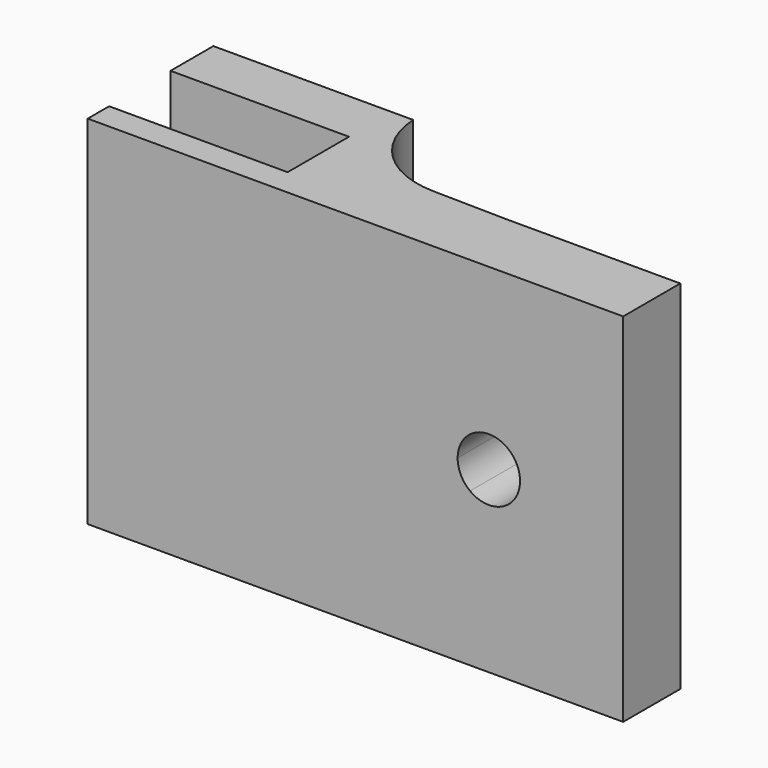
from build123d import *

# Parameters (mm, degrees)
F1_DEPTH    = 20
F2_T1_DEPTH = 20
F4_DEPTH    = 25


# Not quite as in the source:
# - a fillet or chamfer that OpenCascade refuses, or shapes differently, is made with other operations: its cross-section is extruded or revolved along the edge and cut away or added


with BuildPart() as f1:
    # F0 (on Top) → F1 (new body)
    with BuildSketch(Plane.XY):
        Polygon((-30, 0), (0, 0), (0, 1.4936865721), (0, 2.9873731442), (0, 4), (-9.7294932483, 4), (-18.8047308475, 4.1669379548), (-18.8047308475, 8.8), (-30, 8.8), (-30, 5.8), (-20, 5.8), (-20, 1.5), (-30, 1.5), align=None)
    extrude(amount=F1_DEPTH)

    # F2: fillet of radius 5 on 2 edges, made by hand

    # F2_s2 → F2_t1 (join)
    with BuildSketch(Plane.XY):
        with BuildLine():
            ThreePointArc((-9.7754687943, 4.0008457149), (-9.7294913038, 4.0002114332), (-9.6835099246, 4))
            Line((-9.6835099246, 4), (-9.7294932483, 4))
            Line((-9.7294932483, 4), (-9.7754687943, 4.0008457149))
        make_face()
        with BuildLine():
            ThreePointArc((-18.8047308475, 8.8), (-17.2821914607, 5.4759203381), (-13.904310341, 4.0767952816))
            Line((-13.904310341, 4.0767952816), (-18.8047308475, 4.1669379548))
            Line((-18.8047308475, 4.1669379548), (-18.8047308475, 8.8))
        make_face()
    extrude(amount=F2_T1_DEPTH)

    # F3 (on face) → F4 (cut)
    with BuildSketch(Plane(origin=(0, 4, 0), x_dir=(-1, 0, 0), z_dir=(0, 1, 0))):
        with BuildLine():
            Line((6.4737138013, 11.3982501667), (7.5260428712, 10))
            Line((7.5260428712, 10), (8.5783719411, 11.3982501667))
            ThreePointArc((8.5783719411, 11.3982501667), (7.5260428712, 11.75), (6.4737138013, 11.3982501667))
        make_face()
        with BuildLine():
            ThreePointArc((6.4737138013, 11.3982501667), (5.7760428712, 10), (6.4737138013, 8.6017498333))
            Line((6.4737138013, 8.6017498333), (7.5260428712, 10))
            Line((7.5260428712, 10), (6.4737138013, 11.3982501667))
        make_face()
        with BuildLine():
            Line((7.5260428712, 10), (6.4737138013, 8.6017498333))
            ThreePointArc((6.4737138013, 8.6017498333), (7.5260428712, 8.25), (8.5783719411, 8.6017498333))
            Line((8.5783719411, 8.6017498333), (7.5260428712, 10))
        make_face()
        with BuildLine():
            Line((8.5783719411, 11.3982501667), (7.5260428712, 10))
            Line((7.5260428712, 10), (8.5783719411, 8.6017498333))
            ThreePointArc((8.5783719411, 8.6017498333), (9.0919413149, 9.2186792823), (9.2760428712, 10))
            ThreePointArc((9.2760428712, 10), (9.0919413149, 10.7813207177), (8.5783719411, 11.3982501667))
        make_face()
    extrude(amount=-F4_DEPTH, mode=Mode.SUBTRACT)


solid = f1.part
